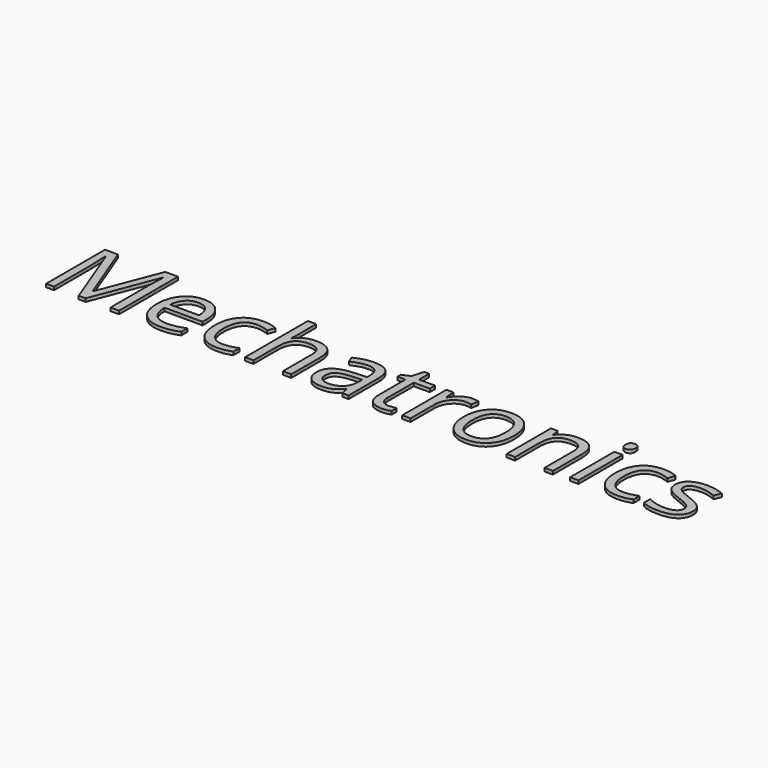
from build123d import *

# Parameters (mm, degrees)
F0_TEXT_SIZE = 9.5028335272
F1_DEPTH     = 0.3


# Not quite as in the source:
# - Text() gives the source's letters only with a copy of the font that has no kerning and outlines rounded to 1/6400 em; it was checked with that copy


with BuildPart() as f1:
    # F0 (on Top) → F1 (new body)
    with BuildSketch(Plane.XY):
        with Locations((-5.3060717769, -3.467564661)):
            Text('Mechatronics', F0_TEXT_SIZE, font='Open Sans', text_align=(TextAlign.LEFT, TextAlign.BOTTOM))
    extrude(amount=F1_DEPTH)


solid = f1.part
